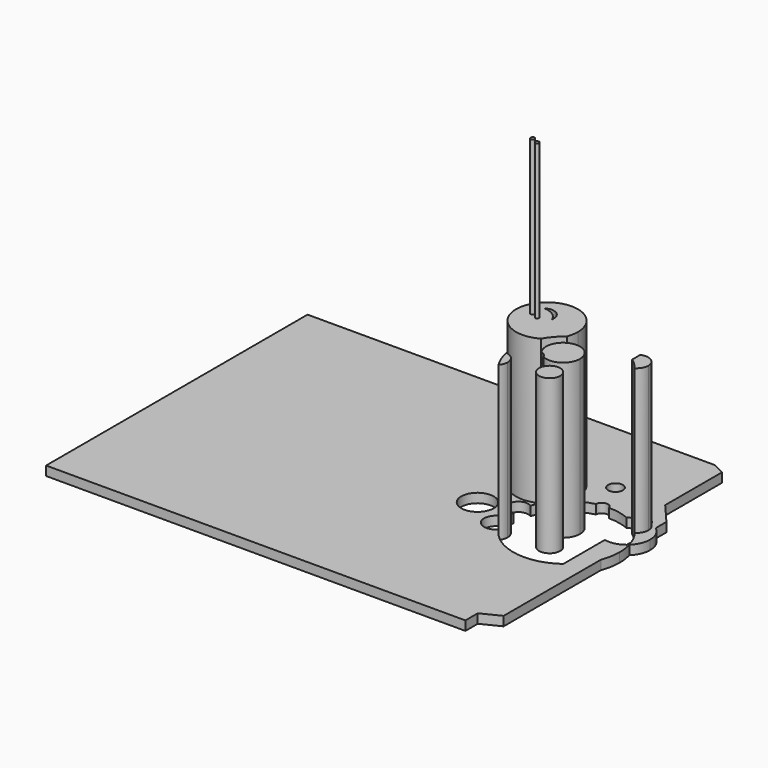
from build123d import *

# Parameters (mm, degrees)
F0_R     = 2.6278375122
F0_R_2   = 1.1924493759
F1_DEPTH = 1.5
F2_DEPTH = 25
F0_R_3   = 1.7150177914
F3_R     = 0.3066007816
F3_R_2   = 0.3212661132
F4_DEPTH = 25
F5_DEPTH = 25


with BuildPart() as f1:
    # F0 (on Top) → F1 (new body)
    with BuildSketch(Plane.XY):
        with BuildLine():
            Line((0, 53), (0, 0))
            Line((0, 0), (68, 0))
            Line((68, 0), (68, 2.5))
            Line((68, 2.5), (68, 19.8288588746))
            ThreePointArc((68, 19.8288588746), (61.3608271995, 18.3286541388), (55.6953940617, 22.1011993122))
            ThreePointArc((55.6953940617, 22.1011993122), (52.4899736453, 22.6494230493), (54.4330548178, 25.2570474218))
            ThreePointArc((54.4330548178, 25.2570474218), (54.3224861562, 26.0713778864), (54.289781951, 26.8925294981))
            ThreePointArc((54.289781951, 26.8925294981), (52.3215154133, 28.6875368607), (54.7834433366, 29.7049038033))
            ThreePointArc((54.7834433366, 29.7049038033), (55.0640203529, 30.4009127933), (55.4039315186, 31.0699511896))
            ThreePointArc((55.4039315186, 31.0699511896), (51.4723174683, 30.611343819), (48.4336038497, 33.1479023744))
            ThreePointArc((48.4336038497, 33.1479023744), (47.8135649338, 34.4460507642), (47.91312779, 35.881224878))
            ThreePointArc((47.91312779, 35.881224878), (53.1376259317, 40.4230819927), (57.9175378005, 35.4154588629))
            ThreePointArc((57.9175378005, 35.4154588629), (57.8328911136, 34.4981199945), (57.5818096181, 33.6117601669))
            ThreePointArc((57.5818096181, 33.6117601669), (59.188306317, 34.613689426), (60.9744599761, 35.241661551))
            ThreePointArc((60.9744599761, 35.241661551), (61.8533262271, 36.1920987658), (62.9249150732, 35.4658521608))
            ThreePointArc((62.9249150732, 35.4658521608), (64.6695885562, 35.2889169352), (66.3426051765, 34.7633629182))
            ThreePointArc((66.3426051765, 34.7633629182), (66.8431977831, 35.1122947347), (67.3941141066, 35.3746638923))
            ThreePointArc((67.3941141066, 35.3746638923), (67.6228355533, 35.8105961465), (68, 36.1269778946))
            Line((68, 36.1269778946), (68, 37))
            Line((68, 37), (68, 40.5))
            Line((68, 40.5), (68, 52))
            Line((68, 52), (66, 53))
            Line((66, 53), (0, 53))
        make_face()
        with Locations((48.9628277719, 26.2474678457)):
            Circle(F0_R, mode=Mode.SUBTRACT)
        with Locations((60.0883662701, 40.3109230101)):
            Circle(F0_R_2, mode=Mode.SUBTRACT)
        with BuildLine():
            Line((68, 19.8288588746), (68, 2.5))
            Line((68, 2.5), (71, 4))
            Line((71, 4), (71, 23.7380924418))
            ThreePointArc((71, 23.7380924418), (69.7845899166, 21.5650774133), (68, 19.8288588746))
        make_face()
        with BuildLine():
            Line((68, 28.2475113294), (68, 19.8288588746))
            ThreePointArc((68, 19.8288588746), (69.7845899166, 21.5650774133), (71, 23.7380924418))
            Line((71, 23.7380924418), (71, 28.9656954726))
            ThreePointArc((71, 28.9656954726), (69.5779809067, 28.2808614275), (68, 28.2475113294))
        make_face()
        with BuildLine():
            Line((71, 28.9656954726), (71, 23.7380924418))
            ThreePointArc((71, 23.7380924418), (71.4265996488, 25.2556300447), (71.5703949044, 26.8254168332))
            ThreePointArc((71.5703949044, 26.8254168332), (71.488644419, 28.0111810019), (71.244939908, 29.1745072318))
            ThreePointArc((71.244939908, 29.1745072318), (71.1247301774, 29.06745007), (71, 28.9656954726))
        make_face()
        Polygon((71, 37), (68, 40.5), (68, 37), align=None)
        with BuildLine():
            Line((71, 29.9127412246), (71, 28.9656954726))
            ThreePointArc((71, 28.9656954726), (71.1247301774, 29.06745007), (71.244939908, 29.1745072318))
            ThreePointArc((71.244939908, 29.1745072318), (71.1307810974, 29.5463817966), (71, 29.9127412246))
        make_face()
        with BuildLine():
            Line((71, 37), (68, 37))
            Line((68, 37), (68, 36.1269778946))
            ThreePointArc((68, 36.1269778946), (69.0584871691, 36.2040282952), (69.8067182705, 35.4513782636))
            ThreePointArc((69.8067182705, 35.4513782636), (70.4317447612, 35.1946578959), (71, 34.8290769271))
            Line((71, 34.8290769271), (71, 37))
        make_face()
        with BuildLine():
            ThreePointArc((70.6559565162, 33.7548259768), (70.4093826923, 32.8295484731), (69.7350587516, 32.1496776527))
            ThreePointArc((69.7350587516, 32.1496776527), (70.4511573148, 31.0784993072), (71, 29.9127412246))
            Line((71, 29.9127412246), (71, 34.8290769271))
            ThreePointArc((71, 34.8290769271), (70.4317447612, 35.1946578959), (69.8067182705, 35.4513782636))
            ThreePointArc((69.8067182705, 35.4513782636), (69.8340876843, 35.3680821722), (69.8556518079, 35.2830979841))
            ThreePointArc((69.8556518079, 35.2830979841), (70.4437735665, 34.6173952428), (70.6559565162, 33.7548259768))
        make_face()
        with BuildLine():
            Line((71, 34.8290769271), (71, 29.9127412246))
            ThreePointArc((71, 29.9127412246), (71.1307810974, 29.5463817966), (71.244939908, 29.1745072318))
            ThreePointArc((71.244939908, 29.1745072318), (72.1215541699, 30.4124106248), (72.4309162817, 31.8973861998))
            ThreePointArc((72.4309162817, 31.8973861998), (72.0540953895, 33.5285155575), (71, 34.8290769271))
        make_face()
    extrude(amount=F1_DEPTH)

    # F0 (on Top) → F2, piece 2 (join)
    with BuildSketch(Plane.XY):
        with BuildLine():
            Line((68, 33.8991143367), (68, 33.8219747917))
            ThreePointArc((68, 33.8219747917), (68.9261149597, 33.0466105336), (69.7350587516, 32.1496776527))
            ThreePointArc((69.7350587516, 32.1496776527), (70.4093826923, 32.8295484731), (70.6559565162, 33.7548259768))
            ThreePointArc((70.6559565162, 33.7548259768), (70.4437735665, 34.6173952428), (69.8556518079, 35.2830979841))
            ThreePointArc((69.8556518079, 35.2830979841), (69.8773872009, 35.1488488132), (69.8846600648, 35.0130461156))
            ThreePointArc((69.8846600648, 35.0130461156), (69.2601125437, 33.9184243125), (68, 33.8991143367))
        make_face()
        with BuildLine():
            Line((68, 35.4348953571), (68, 33.8991143367))
            ThreePointArc((68, 33.8991143367), (69.2601125437, 33.9184243125), (69.8846600648, 35.0130461156))
            ThreePointArc((69.8846600648, 35.0130461156), (69.8773872009, 35.1488488132), (69.8556518079, 35.2830979841))
            ThreePointArc((69.8556518079, 35.2830979841), (69.3915424263, 35.5164301392), (68.8809966916, 35.6122657564))
            ThreePointArc((68.8809966916, 35.6122657564), (68.4296211931, 35.5776072464), (68, 35.4348953571))
        make_face()
        with BuildLine():
            ThreePointArc((55.4039315186, 31.0699511896), (56.3686096023, 32.4473252198), (57.5818096181, 33.6117601669))
            ThreePointArc((57.5818096181, 33.6117601669), (57.8328911136, 34.4981199945), (57.9175378005, 35.4154588629))
            ThreePointArc((57.9175378005, 35.4154588629), (53.1376259317, 40.4230819927), (47.91312779, 35.881224878))
            ThreePointArc((47.91312779, 35.881224878), (48.9153694852, 37.2508061123), (50.5214999846, 37.7990633442))
            ThreePointArc((50.5214999846, 37.7990633442), (52.2965293748, 37.9289651674), (53.2236828127, 36.4097580314))
            ThreePointArc((53.2236828127, 36.4097580314), (53.2154349825, 36.2420960388), (53.1907711372, 36.0760530769))
            ThreePointArc((53.1907711372, 36.0760530769), (53.3578818186, 35.5365305334), (53.414337444, 34.9745489348))
            ThreePointArc((53.414337444, 34.9745489348), (51.5618234293, 32.3219867398), (48.4336038497, 33.1479023744))
            ThreePointArc((48.4336038497, 33.1479023744), (51.4723174683, 30.611343819), (55.4039315186, 31.0699511896))
        make_face()
        with BuildLine():
            ThreePointArc((47.91312779, 35.881224878), (47.9799292355, 34.4777296591), (48.4336038497, 33.1479023744))
            ThreePointArc((48.4336038497, 33.1479023744), (51.5618234293, 32.3219867398), (53.414337444, 34.9745489348))
            ThreePointArc((53.414337444, 34.9745489348), (53.3578818186, 35.5365305334), (53.1907711372, 36.0760530769))
            ThreePointArc((53.1907711372, 36.0760530769), (50.5890162075, 34.9745489348), (50.5214999846, 37.7990633442))
            ThreePointArc((50.5214999846, 37.7990633442), (48.9153694852, 37.2508061123), (47.91312779, 35.881224878))
        make_face()
        with BuildLine():
            ThreePointArc((53.1907711372, 36.0760530769), (52.1212637564, 37.3482922946), (50.5214999846, 37.7990633442))
            ThreePointArc((50.5214999846, 37.7990633442), (50.5890162075, 34.9745489348), (53.1907711372, 36.0760530769))
        make_face()
    extrude(amount=F2_DEPTH)

    # F3 (on face) → F4 (join)
    with BuildSketch(Plane.XY.offset(25)):
        with Locations((51.3830035925, 35.3216975927)):
            Circle(F3_R)
        with Locations((50.2388849854, 35.8146764338)):
            Circle(F3_R_2)
    extrude(amount=-F4_DEPTH)

    # F3 (on face) → F5 (join)
    with BuildSketch(Plane.XY.offset(25)):
        with Locations((51.3830035925, 35.3216975927)):
            Circle(F3_R)
        with Locations((50.2388849854, 35.8146764338)):
            Circle(F3_R_2)
    extrude(amount=F5_DEPTH)


with BuildPart() as f2:
    # F0 (on Top) → F2 (new body)
    with BuildSketch(Plane.XY):
        with BuildLine():
            ThreePointArc((54.4330548178, 25.2570474218), (54.9075139378, 23.6164391663), (55.6953940617, 22.1011993122))
            ThreePointArc((55.6953940617, 22.1011993122), (56.0458256446, 22.686515355), (56.1678403419, 23.3577154577))
            ThreePointArc((56.1678403419, 23.3577154577), (55.668870425, 24.6438863954), (54.4330548178, 25.2570474218))
        make_face()
    extrude(amount=F2_DEPTH)


with BuildPart() as f2b:
    # F0 (on Top) → F2, piece 3 (new body)
    with BuildSketch(Plane.XY):
        with BuildLine():
            ThreePointArc((57.7444498964, 28.2469801579), (58.3749807915, 27.924921367), (58.7896853725, 27.3510649521))
            ThreePointArc((58.7896853725, 27.3510649521), (61.4423382614, 27.4885625868), (62.7305394701, 29.8114940524))
            ThreePointArc((62.7305394701, 29.8114940524), (59.1721797268, 32.4243848348), (57.7444498964, 28.2469801579))
        make_face()
    extrude(amount=F2_DEPTH)


with BuildPart() as f2c:
    # F0 (on Top) → F2, piece 4 (new body)
    with BuildSketch(Plane.XY):
        with Locations((61.9667060673, 24.6099419892)):
            Circle(F0_R_3)
    extrude(amount=F2_DEPTH)


solid = Compound([f1.part, f2.part, f2b.part, f2c.part])
